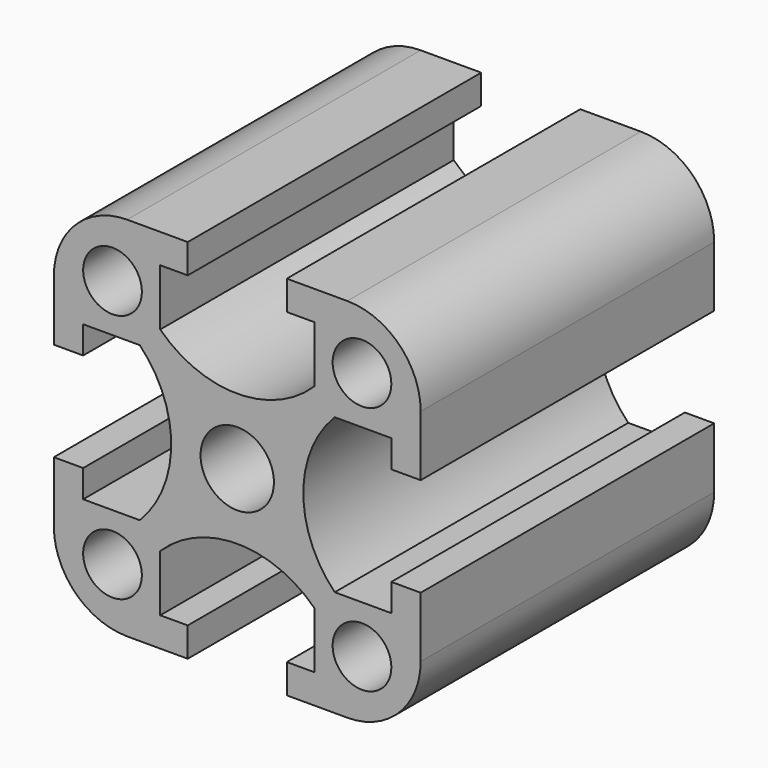
from build123d import *

# Parameters (mm, degrees)
F0_R     = 2
F0_R_2   = 2.5
F2_DEPTH = 25


# Not quite as in the source:
# - ends of sketch curves that miss each other by under 0.0002 mm in the source are joined


with BuildPart() as f2:
    # F0 (on Front) → F2 (new body)
    with BuildSketch(Plane.XZ):
        with BuildLine():
            ThreePointArc((5.2500001607, 6.6439288361), (0, 4.5), (-5.2500001607, 6.6439288361))
            Line((-5.2500001607, 6.6439288361), (-5.25, 10.5))
            Line((-5.25, 10.5), (-3.375, 10.5))
            Line((-3.375, 10.5), (-3.375, 12.5))
            Line((-3.375, 12.5), (-7.5, 12.5))
            ThreePointArc((-7.5, 12.5), (-11.0355339059, 11.0355339059), (-12.5, 7.5))
            Line((-12.5, 7.5), (-12.5, 3.375))
            Line((-12.5, 3.375), (-10.5, 3.375))
            Line((-10.5, 3.375), (-10.5, 5.25))
            Line((-10.5, 5.25), (-6.643929, 5.25))
            ThreePointArc((-6.643929, 5.25), (-4.5, 0), (-6.6439288361, -5.2500001607))
            Line((-6.6439288361, -5.2500001607), (-10.5, -5.25))
            Line((-10.5, -5.25), (-10.5, -3.375))
            Line((-10.5, -3.375), (-12.5, -3.375))
            Line((-12.5, -3.375), (-12.5, -7.5))
            ThreePointArc((-12.5, -7.5), (-11.0355339059, -11.0355339059), (-7.5, -12.5))
            Line((-7.5, -12.5), (-3.375, -12.5))
            Line((-3.375, -12.5), (-3.375, -10.5))
            Line((-3.375, -10.5), (-5.25, -10.5))
            Line((-5.25, -10.5), (-5.25, -6.643929))
            ThreePointArc((-5.25, -6.643929), (0, -4.5), (5.2500001607, -6.6439288361))
            Line((5.2500001607, -6.6439288361), (5.25, -10.5))
            Line((5.25, -10.5), (3.375, -10.5))
            Line((3.375, -10.5), (3.375, -12.5))
            Line((3.375, -12.5), (7.5, -12.5))
            ThreePointArc((7.5, -12.5), (11.0355339059, -11.0355339059), (12.5, -7.5))
            Line((12.5, -7.5), (12.5, -3.375))
            Line((12.5, -3.375), (10.5, -3.375))
            Line((10.5, -3.375), (10.5, -5.25))
            Line((10.5, -5.25), (6.643929, -5.25))
            ThreePointArc((6.643929, -5.25), (4.5, 0), (6.6439288361, 5.2500001607))
            Line((6.6439288361, 5.2500001607), (10.5, 5.25))
            Line((10.5, 5.25), (10.5, 3.375))
            Line((10.5, 3.375), (12.5, 3.375))
            Line((12.5, 3.375), (12.5, 7.5))
            ThreePointArc((12.5, 7.5), (11.0355339059, 11.0355339059), (7.5, 12.5))
            Line((7.5, 12.5), (3.375, 12.5))
            Line((3.375, 12.5), (3.375, 10.5))
            Line((3.375, 10.5), (5.25, 10.5))
            Line((5.25, 10.5), (5.2500001607, 6.6439288361))
        make_face()
        with Locations((-8.5, -8.5)):
            Circle(F0_R, mode=Mode.SUBTRACT)
        with Locations((8.5, -8.5)):
            Circle(F0_R, mode=Mode.SUBTRACT)
        with Locations((-8.5, 8.5)):
            Circle(F0_R, mode=Mode.SUBTRACT)
        Circle(F0_R_2, mode=Mode.SUBTRACT)
        with Locations((8.5, 8.5)):
            Circle(F0_R, mode=Mode.SUBTRACT)
    extrude(amount=F2_DEPTH)


solid = f2.part
